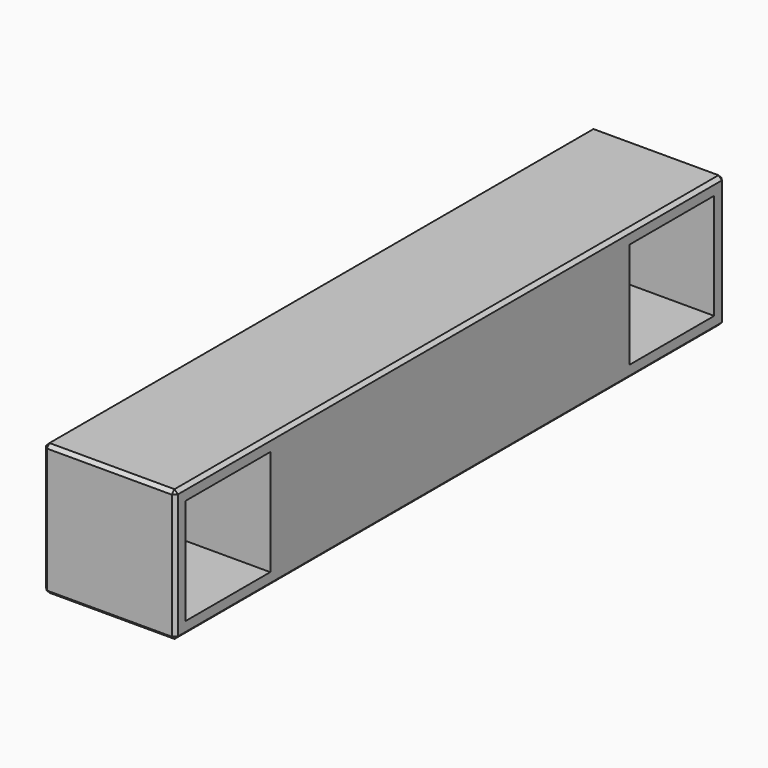
from build123d import *

# Parameters (mm, degrees)
F0_W     = 19.2
F0_H     = 100
F1_DEPTH = 19.2
F2_W     = 15.4
F2_H     = 15.4
F3_DEPTH = 18
F4_SIZE  = 0.5


# Not quite as in the source:
# - a pattern or mirror of a feature is missing from the dataset's text; its kind, count and spacing are read off the source's solid


with BuildPart() as f1:
    # F0 (on Top) → F1 (new body)
    with BuildSketch(Plane.XY):
        Rectangle(F0_W, F0_H)
    extrude(amount=F1_DEPTH)

    # F2 (on face) → F3 (cut)
    with BuildSketch(Plane.YZ.offset(9.6)):
        with Locations((-40.4, 9.6)):
            Rectangle(F2_W, F2_H)
    f3 = extrude(amount=-F3_DEPTH, mode=Mode.SUBTRACT)

    # F3_copies: F3 across plane
    add(f3.mirror(Plane.ZX), mode=Mode.SUBTRACT)

    # F4
    f4_edges = [f1.edges().sort_by_distance(p)[0] for p in [
        (-9.6, 50, 9.6),
        (-9.6, -50, 9.6),
        (-9.6, 0, 0),
        (-9.6, 0, 19.2),
        (0, -50, 19.2),
        (9.6, 0, 19.2),
        (0, 50, 19.2),
        (9.6, -50, 9.6),
        (0, -50, 0),
        (9.6, 0, 0),
        (0, 50, 0),
        (9.6, 50, 9.6),
    ]]
    chamfer(f4_edges, length=F4_SIZE)


solid = f1.part
